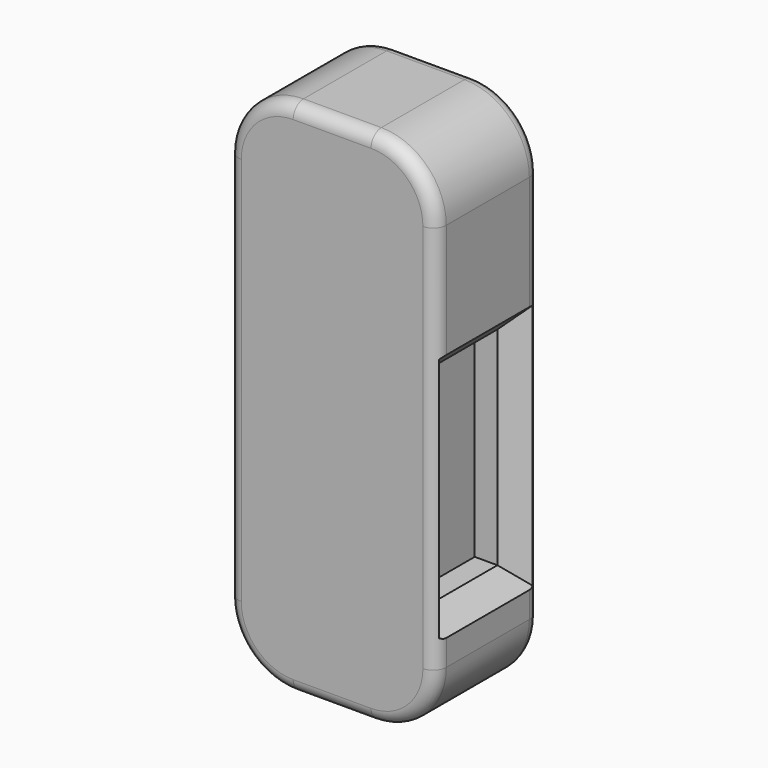
from build123d import *

# Parameters (mm, degrees)
F1_DEPTH     = 31.75
F2_R         = 3.175
F3_W         = 19.05
F3_H         = 50.8
F4_DEPTH     = 10.6367849431
F5_T4_DEPTH  = 76.9282991577
F5_T10_DEPTH = 45.1782991577
F5_T16_DEPTH = 45.1782991577
F5_T22_DEPTH = 76.9282991577


# Not quite as in the source:
# - a fillet or chamfer that OpenCascade refuses, or shapes differently, is made with other operations: its cross-section is extruded or revolved along the edge and cut away or added


with BuildPart() as f1:
    # F0 (on Front) → F1 (new body)
    with BuildSketch(Plane.XZ):
        with BuildLine():
            Line((-5.2392150569, 71.7959681749), (-24.2892150569, 71.7959681749))
            ThreePointArc((-24.2892150569, 71.7959681749), (-35.5145352082, 67.1462883263), (-40.1642150569, 55.9209681749))
            Line((-40.1642150569, 55.9209681749), (-40.1642150569, -39.3290318251))
            ThreePointArc((-40.1642150569, -39.3290318251), (-35.5145352082, -50.5543519764), (-24.2892150569, -55.2040318251))
            Line((-24.2892150569, -55.2040318251), (-5.2392150569, -55.2040318251))
            ThreePointArc((-5.2392150569, -55.2040318251), (5.9861050945, -50.5543519764), (10.6357849431, -39.3290318251))
            Line((10.6357849431, -39.3290318251), (10.6357849431, 55.9209681749))
            ThreePointArc((10.6357849431, 55.9209681749), (5.9861050945, 67.1462883263), (-5.2392150569, 71.7959681749))
        make_face()
    extrude(amount=F1_DEPTH)

    # F2
    f2_edges = [f1.edges().sort_by_distance(p)[0] for p in [
        (-24.289215, -15.875, -55.204032),
        (-5.239215, -15.875, -55.204032),
        (-14.764215, 0, -55.204032),
        (-14.764215, -31.75, -55.204032),
        (-5.239215, -15.875, 71.795968),
        (-24.289215, -15.875, 71.795968),
        (-14.764215, 0, 71.795968),
        (-14.764215, -31.75, 71.795968),
        (10.635785, 0, 8.295968),
        (10.635785, -31.75, 8.295968),
        (5.986105, 0, 67.146288),
        (5.986105, -31.75, 67.146288),
        (-35.514535, 0, 67.146288),
        (-35.514535, -31.75, 67.146288),
        (-40.164215, 0, 8.295968),
        (-40.164215, -31.75, 8.295968),
        (-35.514535, 0, -50.554352),
        (-35.514535, -31.75, -50.554352),
        (5.986105, 0, -50.554352),
        (5.986105, -31.75, -50.554352),
    ]]
    fillet(f2_edges, radius=F2_R)

    # F3 (on Right) → F4 (cut, through all)
    with BuildSketch(Plane.YZ):
        with Locations((-16.1061841063, -2.5141499803)):
            Rectangle(F3_W, F3_H)
    extrude(amount=F4_DEPTH, mode=Mode.SUBTRACT)

    # F5: chamfer of 5.08 on 4 edges, made by hand


with BuildPart() as f5_tool2:
    # F5_s3 → F5_t4 (new body)
    with BuildSketch(Plane.XY.offset(35.9499995986)):
        Polygon((10.6357849431, -30.7111841063), (5.5557849431, -25.6311841063), (10.6357849431, -25.6311841063), align=None)
    extrude(amount=-F5_T4_DEPTH)

    split(bisect_by=Plane(origin=(-11.1791825186, 0, -11.1791825186), x_dir=(0, 1, 0), z_dir=(0.7071067812, 0, 0.7071067812)), keep=Keep.TOP)

    split(bisect_by=Plane(origin=(-8.6650325383, 0, 8.6650325383), x_dir=(0, 1, 0), z_dir=(0.7071067812, 0, -0.7071067812)), keep=Keep.TOP)


with BuildPart() as f1_1:
    add(f1.part)

    # F5_t1: cut F5_tool2
    add(f5_tool2.part, mode=Mode.SUBTRACT)


with BuildPart() as f5_tool8:
    # F5_s9 → F5_t10 (new body)
    with BuildSketch(Plane.XZ.offset(-6.4829654725)):
        Polygon((10.6357849431, 27.9658500197), (5.5557849431, 22.8858500197), (10.6357849431, 22.8858500197), align=None)
    extrude(amount=F5_T10_DEPTH)

    split(bisect_by=Plane(origin=(-10.0376995816, -10.0376995816, 0), x_dir=(0, 0, 1), z_dir=(0.7071067812, 0.7071067812, 0)), keep=Keep.TOP)

    split(bisect_by=Plane(origin=(6.0684845247, -6.0684845247, 0), x_dir=(0, 0, 1), z_dir=(0.7071067812, -0.7071067812, 0)), keep=Keep.TOP)


with BuildPart() as f1_2:
    add(f1_1.part)

    # F5_t7: cut F5_tool8
    add(f5_tool8.part, mode=Mode.SUBTRACT)


with BuildPart() as f5_tool14:
    # F5_s15 → F5_t16 (new body)
    with BuildSketch(Plane.XZ.offset(38.6953336852)):
        Polygon((10.6357849431, -32.9941499803), (5.5557849431, -27.9141499803), (10.6357849431, -27.9141499803), align=None)
    extrude(amount=-F5_T16_DEPTH)

    split(bisect_by=Plane(origin=(-10.0376995816, -10.0376995816, 0), x_dir=(0, 0, 1), z_dir=(0.7071067812, 0.7071067812, 0)), keep=Keep.TOP)

    split(bisect_by=Plane(origin=(6.0684845247, -6.0684845247, 0), x_dir=(0, 0, 1), z_dir=(0.7071067812, -0.7071067812, 0)), keep=Keep.TOP)


with BuildPart() as f1_3:
    add(f1_2.part)

    # F5_t13: cut F5_tool14
    add(f5_tool14.part, mode=Mode.SUBTRACT)


with BuildPart() as f5_tool20:
    # F5_s21 → F5_t22 (new body)
    with BuildSketch(Plane.XY.offset(-40.9782995592)):
        Polygon((10.6357849431, -1.5011841063), (5.5557849431, -6.5811841063), (10.6357849431, -6.5811841063), align=None)
    extrude(amount=F5_T22_DEPTH)

    split(bisect_by=Plane(origin=(-11.1791825186, 0, -11.1791825186), x_dir=(0, 1, 0), z_dir=(0.7071067812, 0, 0.7071067812)), keep=Keep.TOP)

    split(bisect_by=Plane(origin=(-8.6650325383, 0, 8.6650325383), x_dir=(0, 1, 0), z_dir=(0.7071067812, 0, -0.7071067812)), keep=Keep.TOP)


with BuildPart() as f1_4:
    add(f1_3.part)

    # F5_t19: cut F5_tool20
    add(f5_tool20.part, mode=Mode.SUBTRACT)


solid = f1_4.part
